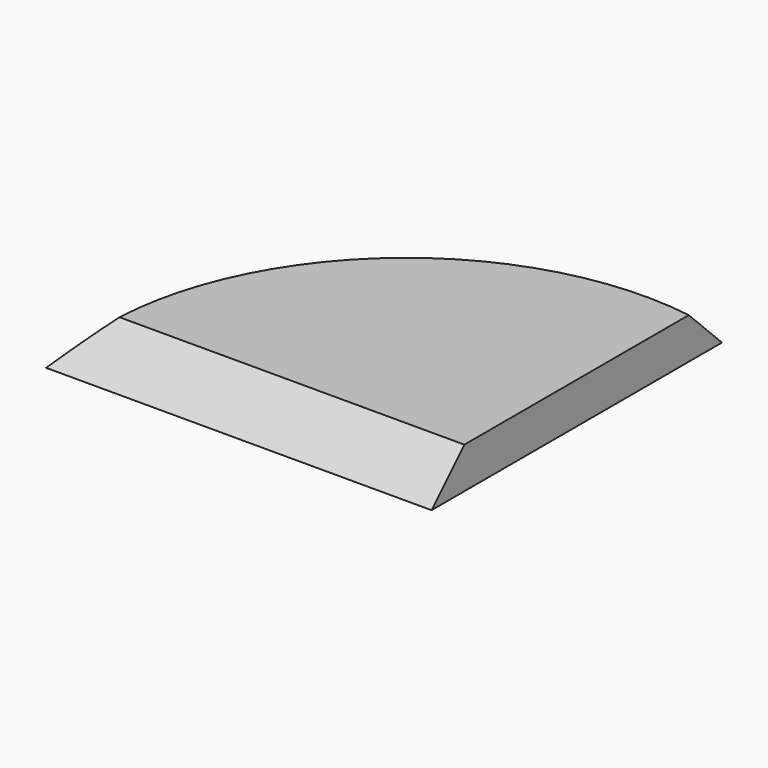
from build123d import *

# Parameters (mm, degrees)
F1_DEPTH = 5.08
F2_SIZE  = 5.07999


# Not quite as in the source:
# - a fillet or chamfer is up to 0.001 mm smaller than in the source, because OpenCascade refuses the exact size


with BuildPart() as f1:
    # F0 (on Top) → F1 (new body)
    with BuildSketch(Plane.XY):
        with BuildLine():
            Line((0, 0), (0, 44.9222251773))
            ThreePointArc((0, 44.9222251773), (-34.5622433169, 33.8350362208), (-47.7024391294, 0))
            Line((-47.7024391294, 0), (0, 0))
        make_face()
    extrude(amount=F1_DEPTH)

    # F2 (size 5.08 in the source; OpenCascade refuses exactly that, so slightly less here)
    f2_edges = [f1.edges().sort_by_distance(p)[0] for p in [
        (-34.562243, 33.835036, 5.08),
        (-23.85122, 0, 5.08),
    ]]
    chamfer(f2_edges, length=F2_SIZE)


solid = f1.part
